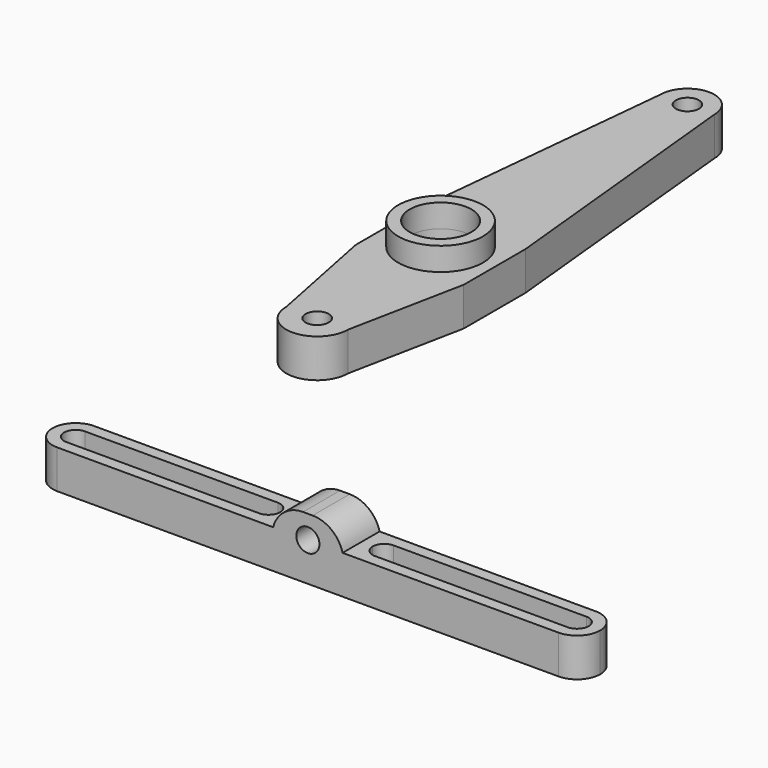
from build123d import *

# Parameters (mm, degrees)
F0_R         = 1.5
F1_DEPTH     = 5
F2_R         = 5.5
F2_R_2       = 4
F3_DEPTH     = 3
F5_DEPTH     = 5
F6_W         = 9
F6_H         = 6
F7_DEPTH     = 3
F8_R         = 1.5
F9_DEPTH     = 25
F10_T1_DEPTH = 25.364916731


# Not quite as in the source:
# - a fillet or chamfer that OpenCascade refuses, or shapes differently, is made with other operations: its cross-section is extruded or revolved along the edge and cut away or added


with BuildPart() as f1:
    # F0 (on Top) → F1 (new body)
    with BuildSketch(Plane.XY):
        with BuildLine():
            ThreePointArc((-48.0446585417, 19.1218993813), (-44.0446585417, 23.1218993813), (-40.0446585417, 19.1218993813))
            Line((-40.0446585417, 19.1218993813), (-37.0446585417, 19.1218993813))
            Line((-37.0446585417, 19.1218993813), (-37.0446585417, 24.1218993813))
            Line((-37.0446585417, 24.1218993813), (-40.5446585417, 59.1218993813))
            ThreePointArc((-40.5446585417, 59.1218993813), (-44.0446585417, 55.6218993813), (-47.5446585417, 59.1218993813))
            Line((-47.5446585417, 59.1218993813), (-51.0446585417, 24.1218993813))
            Line((-51.0446585417, 24.1218993813), (-51.0446585417, 19.1218993813))
            Line((-51.0446585417, 19.1218993813), (-48.0446585417, 19.1218993813))
        make_face()
        with BuildLine():
            Line((-37.0446585417, 19.1218993813), (-40.0446585417, 19.1218993813))
            ThreePointArc((-40.0446585417, 19.1218993813), (-44.0446585417, 15.1218993813), (-48.0446585417, 19.1218993813))
            Line((-48.0446585417, 19.1218993813), (-51.0446585417, 19.1218993813))
            Line((-51.0446585417, 19.1218993813), (-51.0446585417, 14.1218993813))
            Line((-51.0446585417, 14.1218993813), (-48.0446585417, -0.8781006187))
            ThreePointArc((-48.0446585417, -0.8781006187), (-44.0446585417, 3.1218993813), (-40.0446585417, -0.8781006187))
            Line((-40.0446585417, -0.8781006187), (-37.0446585417, 14.1218993813))
            Line((-37.0446585417, 14.1218993813), (-37.0446585417, 19.1218993813))
        make_face()
        with BuildLine():
            ThreePointArc((-48.0446585417, -0.8781006187), (-44.0446585417, -4.8781006187), (-40.0446585417, -0.8781006187))
            ThreePointArc((-40.0446585417, -0.8781006187), (-44.0446585417, 3.1218993813), (-48.0446585417, -0.8781006187))
        make_face()
        with Locations((-44.0446585417, -0.8781006187)):
            Circle(F0_R, mode=Mode.SUBTRACT)
        with BuildLine():
            ThreePointArc((-47.5446585417, 59.1218993813), (-44.0446585417, 55.6218993813), (-40.5446585417, 59.1218993813))
            ThreePointArc((-40.5446585417, 59.1218993813), (-44.0446585417, 62.6218993813), (-47.5446585417, 59.1218993813))
        make_face()
        with Locations((-44.0446585417, 59.1218993813)):
            Circle(F0_R, mode=Mode.SUBTRACT)
    extrude(amount=F1_DEPTH)

    # F2 (on face) → F3 (join)
    with BuildSketch(Plane.XY.offset(5)):
        with Locations((-44.0446585417, 19.1218993813)):
            Circle(F2_R)
        with Locations((-44.0446585417, 19.1218993813)):
            Circle(F2_R_2, mode=Mode.SUBTRACT)
    extrude(amount=F3_DEPTH)


with BuildPart() as f5:
    # F4 (on Top) → F5 (new body)
    with BuildSketch(Plane.XY):
        with BuildLine():
            ThreePointArc((-46.904212172, -33.4348478615), (-45.404212172, -33.8367716502), (-44.3061359607, -34.9348478615))
            Line((-44.3061359607, -34.9348478615), (-21.904212172, -34.9348478615))
            ThreePointArc((-21.904212172, -34.9348478615), (-20.8435520003, -35.3741876897), (-20.404212172, -36.4348478615))
            Line((-20.404212172, -36.4348478615), (-8.404212172, -36.4348478615))
            ThreePointArc((-8.404212172, -36.4348478615), (-7.9648723438, -35.3741876897), (-6.904212172, -34.9348478615))
            Line((-6.904212172, -34.9348478615), (15.4977116166, -34.9348478615))
            ThreePointArc((15.4977116166, -34.9348478615), (16.595787828, -33.8367716502), (18.095787828, -33.4348478615))
            Line((18.095787828, -33.4348478615), (-46.904212172, -33.4348478615))
        make_face()
        with BuildLine():
            Line((-21.904212172, -37.9348478615), (-44.3061359607, -37.9348478615))
            ThreePointArc((-44.3061359607, -37.9348478615), (-45.404212172, -39.0329240729), (-46.904212172, -39.4348478615))
            Line((-46.904212172, -39.4348478615), (18.095787828, -39.4348478615))
            ThreePointArc((18.095787828, -39.4348478615), (16.595787828, -39.0329240729), (15.4977116166, -37.9348478615))
            Line((15.4977116166, -37.9348478615), (-6.904212172, -37.9348478615))
            ThreePointArc((-6.904212172, -37.9348478615), (-7.9648723438, -37.4955080333), (-8.404212172, -36.4348478615))
            Line((-8.404212172, -36.4348478615), (-20.404212172, -36.4348478615))
            ThreePointArc((-20.404212172, -36.4348478615), (-20.8435520003, -37.4955080333), (-21.904212172, -37.9348478615))
        make_face()
        with BuildLine():
            ThreePointArc((-46.904212172, -37.9348478615), (-48.404212172, -36.4348478615), (-46.904212172, -34.9348478615))
            Line((-46.904212172, -34.9348478615), (-44.3061359607, -34.9348478615))
            ThreePointArc((-44.3061359607, -34.9348478615), (-45.404212172, -33.8367716502), (-46.904212172, -33.4348478615))
            ThreePointArc((-46.904212172, -33.4348478615), (-49.904212172, -36.4348478615), (-46.904212172, -39.4348478615))
            ThreePointArc((-46.904212172, -39.4348478615), (-45.404212172, -39.0329240729), (-44.3061359607, -37.9348478615))
            Line((-44.3061359607, -37.9348478615), (-46.904212172, -37.9348478615))
        make_face()
        with BuildLine():
            ThreePointArc((21.095787828, -36.4348478615), (20.2171081715, -34.313527518), (18.095787828, -33.4348478615))
            ThreePointArc((18.095787828, -33.4348478615), (16.595787828, -33.8367716502), (15.4977116166, -34.9348478615))
            Line((15.4977116166, -34.9348478615), (18.095787828, -34.9348478615))
            ThreePointArc((18.095787828, -34.9348478615), (19.1564479997, -35.3741876897), (19.595787828, -36.4348478615))
            ThreePointArc((19.595787828, -36.4348478615), (19.1564479997, -37.4955080333), (18.095787828, -37.9348478615))
            Line((18.095787828, -37.9348478615), (15.4977116166, -37.9348478615))
            ThreePointArc((15.4977116166, -37.9348478615), (16.595787828, -39.0329240729), (18.095787828, -39.4348478615))
            ThreePointArc((18.095787828, -39.4348478615), (20.2171081715, -38.5561682051), (21.095787828, -36.4348478615))
        make_face()
    extrude(amount=F5_DEPTH)

    # F6 (on face) → F7 (join)
    with BuildSketch(Plane.XY.offset(5)):
        with Locations((-14.404212172, -36.4348478615)):
            Rectangle(F6_W, F6_H)
    extrude(amount=F7_DEPTH)

    # F8 (on face) → F9 (cut)
    with BuildSketch(Plane.XZ.offset(39.4348478615)):
        with Locations((-14.404212172, 5)):
            Circle(F8_R)
    extrude(amount=-F9_DEPTH, mode=Mode.SUBTRACT)

    # F10: fillet of radius 4 on 2 edges, made by hand

    # F10_s2 → F10_t1 (cut)
    with BuildSketch(Plane.XZ.offset(23.752389496)):
        with BuildLine():
            ThreePointArc((-15.0312288258, 8), (-17.4807185686, 7.1622776602), (-18.904212172, 5))
            Line((-18.904212172, 5), (-18.904212172, 8))
            Line((-18.904212172, 8), (-15.0312288258, 8))
        make_face()
        with BuildLine():
            ThreePointArc((-9.904212172, 5), (-11.3277057755, 7.1622776602), (-13.7771955183, 8))
            Line((-13.7771955183, 8), (-9.904212172, 8))
            Line((-9.904212172, 8), (-9.904212172, 5))
        make_face()
    extrude(amount=F10_T1_DEPTH, mode=Mode.SUBTRACT)


solid = Compound([f1.part, f5.part])
